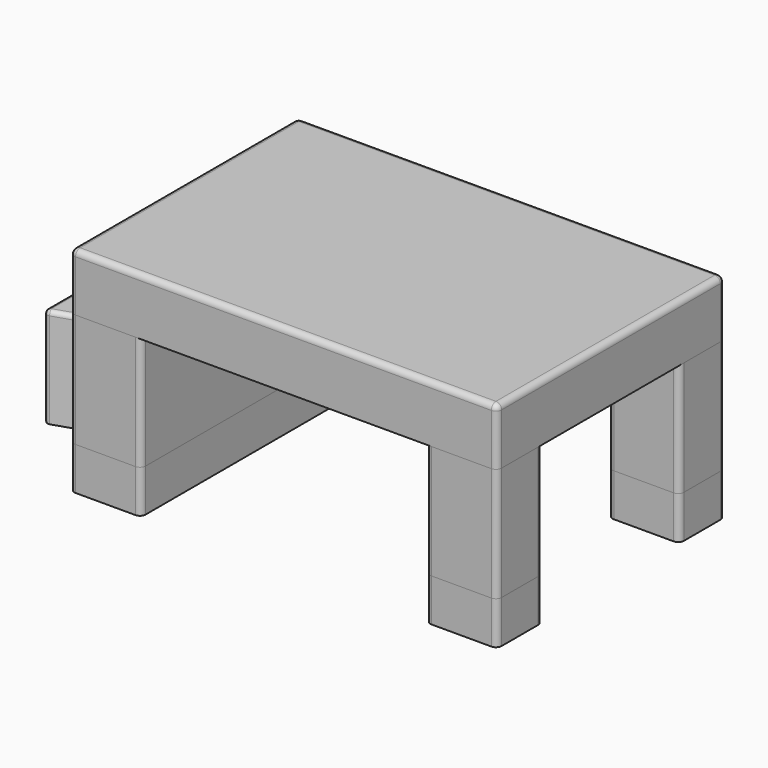
from build123d import *

# Parameters (mm, degrees)
F1_DEPTH = 16
F0_W     = 10
F0_H     = 8
F2_DEPTH = 14
F3_W     = 60
F3_H     = 40
F4_DEPTH = 3
F5_DEPTH = 8
F6_DEPTH = 6
F7_R     = 0.6
F8_R     = 0.8
F8_2_R   = 0.8
F8_3_R   = 0.8
F8_4_R   = 0.8
F8_5_R   = 0.8
F8_6_R   = 0.8
F8_7_R   = 0.8
F8_8_R   = 0.8


# Not quite as in the source:
# - a feature names something its author has since deleted; it is built from what else it names


with BuildPart() as f1:
    # F0 (on Top) → F1 (new body)
    with BuildSketch(Plane.XY):
        Polygon((-20, 20), (-30, 20), (-30, 16.6), (-30, 11.4), (-30, -11.4), (-30, -16.6), (-30, -20), (-20, -20), align=None)
    extrude(amount=F1_DEPTH)

    # F0 (on Top) → F2 (join)
    with BuildSketch(Plane.XY):
        Polygon((-30, -16.6), (-30, -11.4), (-35.2, -9.7), (-35.2, -18.3), align=None)
        Polygon((-30, 11.4), (-30, 16.6), (-35.2, 18.3), (-35.2, 9.7), align=None)
    extrude(amount=F2_DEPTH)

    # F7
    f7_edges = [f1.edges().sort_by_distance(p)[0] for p in [
        (-35.2, 18.3, 7),
        (-35.2, 9.7, 7),
        (-35.2, 14, 0),
        (-35.2, 14, 14),
        (-30, 14, 14),
        (-32.6, 17.45, 14),
        (-32.6, 10.55, 14),
        (-32.6, -10.55, 14),
        (-35.2, -14, 14),
        (-32.6, -17.45, 14),
        (-30, -14, 14),
        (-35.2, -9.7, 7),
        (-35.2, -18.3, 7),
        (-35.2, -14, 0),
        (-30, 16.6, 7),
        (-30, 11.4, 7),
        (-30, -11.4, 7),
        (-30, -16.6, 7),
    ]]
    fillet(f7_edges, radius=F7_R)

    # F8
    f8_edges = [f1.edges().sort_by_distance(p)[0] for p in [
        (-20, 20, 8),
        (-30, 20, 8),
        (-30, -20, 8),
        (-20, -20, 8),
    ]]
    fillet(f8_edges, radius=F8_R)


with BuildPart() as f1b:
    # F0 (on Top) → F1, piece 2 (new body)
    with BuildSketch(Plane.XY):
        with Locations((25, 16)):
            Rectangle(F0_W, F0_H)
    extrude(amount=F1_DEPTH)

    # F8#2
    f8_2_edges = [f1b.edges().sort_by_distance(p)[0] for p in [
        (30, 20, 8),
        (30, 12, 8),
        (20, 12, 8),
        (20, 20, 8),
    ]]
    fillet(f8_2_edges, radius=F8_2_R)


with BuildPart() as f1c:
    # F0 (on Top) → F1, piece 3 (new body)
    with BuildSketch(Plane.XY):
        with Locations((25, -16)):
            Rectangle(F0_W, F0_H)
    extrude(amount=F1_DEPTH)

    # F8#3
    f8_3_edges = [f1c.edges().sort_by_distance(p)[0] for p in [
        (30, -20, 8),
        (30, -12, 8),
        (20, -20, 8),
        (20, -12, 8),
    ]]
    fillet(f8_3_edges, radius=F8_3_R)


with BuildPart() as f4:
    # F3 (on face) → F4 (new body)
    with BuildSketch(Plane.XY.offset(16)):
        Rectangle(F3_W, F3_H)
    extrude(amount=F4_DEPTH)

    # F8#4
    f8_4_edges = [f4.edges().sort_by_distance(p)[0] for p in [
        (30, 20, 17.5),
        (30, -20, 17.5),
        (-30, 20, 17.5),
        (-30, -20, 17.5),
    ]]
    fillet(f8_4_edges, radius=F8_4_R)


with BuildPart() as f5:
    # F3 (on face) → F5 (new body)
    with BuildSketch(Plane.XY.offset(16)):
        Rectangle(F3_W, F3_H)
    extrude(amount=F5_DEPTH)

    # F8#5
    f8_5_edges = [f5.edges().sort_by_distance(p)[0] for p in [
        (0, 20, 16),
        (0, 20, 24),
        (30, 20, 20),
        (30, 0, 24),
        (0, -20, 24),
        (-30, 0, 24),
        (-30, -20, 20),
        (-30, 20, 20),
        (30, -20, 20),
    ]]
    fillet(f8_5_edges, radius=F8_5_R)


with BuildPart() as f6:
    # F0 (on Top) → F6 (new body)
    with BuildSketch(Plane.XY):
        Polygon((-20, 20), (-30, 20), (-30, 16.6), (-30, 11.4), (-30, -11.4), (-30, -16.6), (-30, -20), (-20, -20), align=None)
    extrude(amount=-F6_DEPTH)

    # F8#6
    f8_6_edges = [f6.edges().sort_by_distance(p)[0] for p in [
        (-20, 20, -3),
        (-30, 20, -3),
        (-30, -20, -3),
        (-20, -20, -3),
    ]]
    fillet(f8_6_edges, radius=F8_6_R)


with BuildPart() as f6b:
    # F0 (on Top) → F6, piece 2 (new body)
    with BuildSketch(Plane.XY):
        with Locations((25, -16)):
            Rectangle(F0_W, F0_H)
    extrude(amount=-F6_DEPTH)

    # F8#7
    f8_7_edges = [f6b.edges().sort_by_distance(p)[0] for p in [
        (30, -20, -3),
        (30, -12, -3),
        (20, -20, -3),
        (20, -12, -3),
    ]]
    fillet(f8_7_edges, radius=F8_7_R)


with BuildPart() as f6c:
    # F0 (on Top) → F6, piece 3 (new body)
    with BuildSketch(Plane.XY):
        with Locations((25, 16)):
            Rectangle(F0_W, F0_H)
    extrude(amount=-F6_DEPTH)

    # F8#8
    f8_8_edges = [f6c.edges().sort_by_distance(p)[0] for p in [
        (30, 20, -3),
        (30, 12, -3),
        (20, 12, -3),
        (20, 20, -3),
    ]]
    fillet(f8_8_edges, radius=F8_8_R)


solid = Compound([f1.part, f1b.part, f1c.part, f4.part, f5.part, f6.part, f6b.part, f6c.part])
